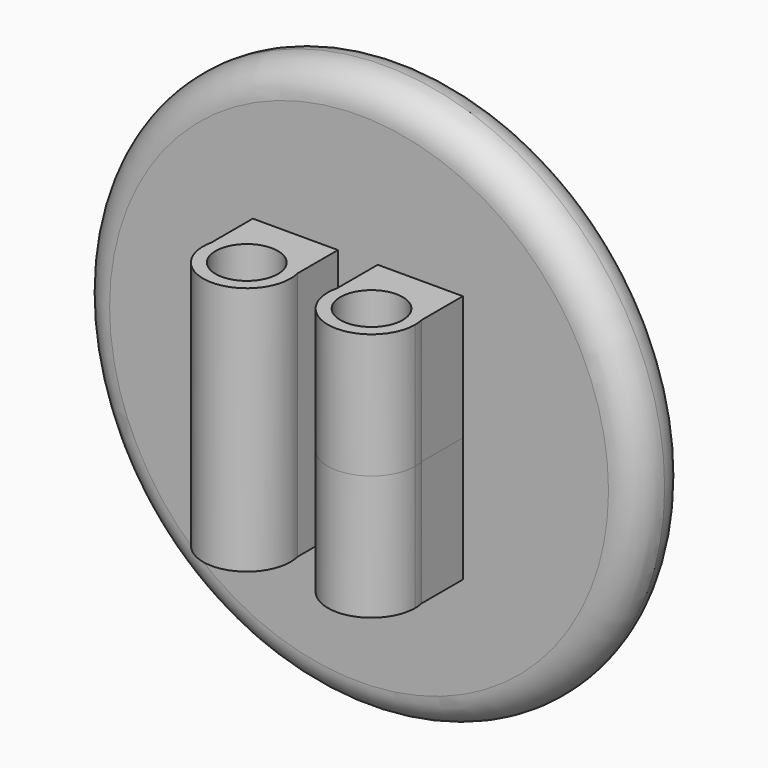
from build123d import *

# Parameters (mm, degrees)
F0_R          = 28.575
F1_DEPTH      = 6.35
F2_R          = 3.17499
F3_R          = 3.175
F4_DEPTH      = 12.7
F4_DEPTH_BACK = 12.7


# Not quite as in the source:
# - a fillet or chamfer is up to 0.001 mm smaller than in the source, because OpenCascade refuses the exact size


with BuildPart() as f1:
    # F0 (on Front) → F1 (new body)
    with BuildSketch(Plane.XZ):
        Circle(F0_R)
    extrude(amount=F1_DEPTH)

    # F2 (radius 3.175 in the source; OpenCascade refuses exactly that, so slightly less here)
    f2_edges = [f1.edges().sort_by_distance(p)[0] for p in [
        (-28.575, -6.35, 0),
        (28.575, -3.175, 0),
        (-28.575, 0, 0),
    ]]
    fillet(f2_edges, radius=F2_R)


with BuildPart() as f4:
    # F3 (on Top) → F4 (new body, two sides)
    with BuildSketch(Plane.XY) as f4_sk:
        with BuildLine():
            ThreePointArc((2.0279974168, -11.6615787604), (5.8271599108, -17.1141435456), (10.795, -12.7))
            ThreePointArc((10.795, -12.7), (10.7691479997, -12.2212976328), (10.691892708, -11.7481635057))
            ThreePointArc((10.691892708, -11.7481635057), (6.3944199707, -8.2552219553), (2.0279974168, -11.6615787604))
        make_face()
        with Locations((6.35, -12.7)):
            Circle(F3_R, mode=Mode.SUBTRACT)
        with BuildLine():
            ThreePointArc((2.0279974168, -11.6615787604), (6.3944199707, -8.2552219553), (10.691892708, -11.7481635057))
            Line((10.691892708, -11.7481635057), (10.691892708, -6.5039667386))
            Line((10.691892708, -6.5039667386), (2.0279974168, -6.5039667386))
            Line((2.0279974168, -6.5039667386), (2.0279974168, -11.6615787604))
        make_face()
    extrude(amount=F4_DEPTH)
    extrude(f4_sk.sketch, amount=-F4_DEPTH_BACK)


with BuildPart() as f4b:
    # F3 (on Top) → F4, piece 2 (new body, two sides)
    with BuildSketch(Plane.XY) as f4_2_sk:
        with BuildLine():
            ThreePointArc((-10.691892708, -11.7481635057), (-6.3944199707, -8.2552219553), (-2.0279974168, -11.6615787604))
            Line((-2.0279974168, -11.6615787604), (-2.0279974168, -6.5039667386))
            Line((-2.0279974168, -6.5039667386), (-10.691892708, -6.5039667386))
            Line((-10.691892708, -6.5039667386), (-10.691892708, -11.7481635057))
        make_face()
        with BuildLine():
            ThreePointArc((-1.905, -12.7), (-1.9358564544, -12.1771599108), (-2.0279974168, -11.6615787604))
            ThreePointArc((-2.0279974168, -11.6615787604), (-6.3944199707, -8.2552219553), (-10.691892708, -11.7481635057))
            ThreePointArc((-10.691892708, -11.7481635057), (-6.8287023672, -17.1191479997), (-1.905, -12.7))
        make_face()
        with Locations((-6.35, -12.7)):
            Circle(F3_R, mode=Mode.SUBTRACT)
    extrude(amount=F4_DEPTH)
    extrude(f4_2_sk.sketch, amount=-F4_DEPTH_BACK)


solid = Compound([f1.part, f4.part, f4b.part])
